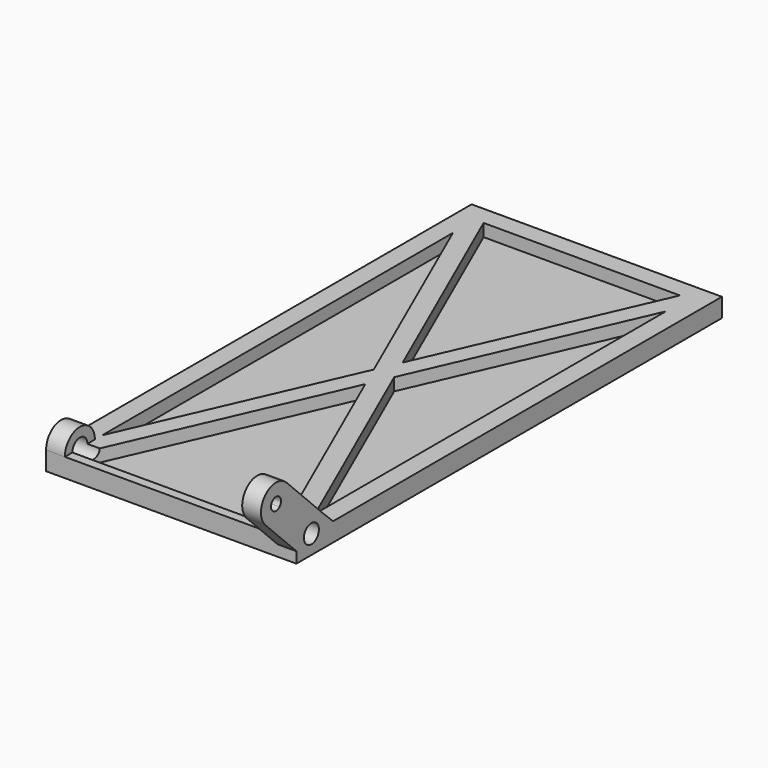
from build123d import *

# Parameters (mm, degrees)
F0_W      = 40
F0_H      = 85
F1_DEPTH  = 1
F2_W      = 3
F2_H      = 3
F3_DEPTH  = 2
F5_DEPTH  = 3
F7_DEPTH  = 3
F9_R      = 1.5
F10_DEPTH = 45


with BuildPart() as f1:
    # F0 (on Top) → F1 (new body)
    with BuildSketch(Plane.XY):
        Rectangle(F0_W, F0_H)
    extrude(amount=F1_DEPTH)

    # F2 (on face) → F3 (join)
    with BuildSketch(Plane.XY.offset(1)):
        Polygon((-17, -42.5), (17, -42.5), (15.6843836329, -39.5), (-15.6843836329, -39.5), align=None)
        Polygon((-17, -39.5), (-17, -42.5), (-15.6843836329, -39.5), align=None)
        with Locations((-18.5, -41)):
            Rectangle(F2_W, F2_H)
        Polygon((15.6843836329, -39.5), (17, -42.5), (17, -39.5), align=None)
        with Locations((18.5, -41)):
            Rectangle(F2_W, F2_H)
        Polygon((17, -35.0301999523), (17, -39.5), (20, -39.5), (20, 39.5), (17, 39.5), (17, 35.0301999523), align=None)
        Polygon((15.6843836329, -39.5), (17, -39.5), (17, -35.0301999523), (1.6378985336, 0), (0, -3.7349000238), align=None)
        Polygon((-15.6843836329, -39.5), (0, -3.7349000238), (-1.6378985336, 0), (-17, -35.0301999523), (-17, -39.5), align=None)
        Polygon((-20, -39.5), (-17, -39.5), (-17, -35.0301999523), (-17, 35.0301999523), (-17, 39.5), (-20, 39.5), align=None)
        Polygon((-1.6378985336, 0), (0, -3.7349000238), (1.6378985336, 0), (0, 3.7349000238), align=None)
        Polygon((-17, 35.0301999523), (-1.6378985336, 0), (0, 3.7349000238), (-15.6843836329, 39.5), (-17, 39.5), align=None)
        Polygon((1.6378985336, 0), (17, 35.0301999523), (17, 39.5), (15.6843836329, 39.5), (0, 3.7349000238), align=None)
        with Locations((-18.5, 41)):
            Rectangle(F2_W, F2_H)
        Polygon((-17, 39.5), (-15.6843836329, 39.5), (-17, 42.5), align=None)
        Polygon((15.6843836329, 39.5), (17, 42.5), (-17, 42.5), (-15.6843836329, 39.5), align=None)
        Polygon((15.6843836329, 39.5), (17, 39.5), (17, 42.5), align=None)
        with Locations((18.5, 41)):
            Rectangle(F2_W, F2_H)
    extrude(amount=F3_DEPTH)

    # F4 (on face) → F5 (join)
    with BuildSketch(Plane.YZ.offset(20)):
        with BuildLine():
            ThreePointArc((-42.5, 3), (-42.2716385975, 4.1480502971), (-41.6213203436, 5.1213203436))
            Line((-41.6213203436, 5.1213203436), (-44.4490675498, 7.9490675498))
            ThreePointArc((-44.4490675498, 7.9490675498), (-46.5442111918, 7.0702264387), (-48.6547486938, 7.9114279791))
            Line((-48.6547486938, 7.9114279791), (-42.5, 1.7572743533))
            Line((-42.5, 1.7572743533), (-42.5, 3))
        make_face()
        with BuildLine():
            Line((-39.5, 3), (-36.5, 3))
            ThreePointArc((-36.5, 3), (-36.7387500509, 4.1728165749), (-37.4169991456, 5.1589598052))
            ThreePointArc((-37.4169991456, 5.1589598052), (-39.5268566208, 5.9998797846), (-41.6213203436, 5.1213203436))
            Line((-41.6213203436, 5.1213203436), (-39.5, 3))
        make_face()
        with BuildLine():
            Line((-42.5, 3), (-39.5, 3))
            Line((-39.5, 3), (-41.6213203436, 5.1213203436))
            ThreePointArc((-41.6213203436, 5.1213203436), (-42.2716385975, 4.1480502971), (-42.5, 3))
        make_face()
        with BuildLine():
            ThreePointArc((-37.4169991456, 5.1589598052), (-36.7387500509, 4.1728165749), (-36.5, 3))
            Line((-36.5, 3), (-35.1793104616, 3))
            Line((-35.1793104616, 3), (-37.4169991456, 5.1589598052))
        make_face()
        with BuildLine():
            ThreePointArc((-41.6213203436, 5.1213203436), (-39.5268566208, 5.9998797846), (-37.4169991456, 5.1589598052))
            Line((-37.4169991456, 5.1589598052), (-44.3843033436, 12.1262640032))
            ThreePointArc((-44.3843033436, 12.1262640032), (-43.7810708304, 11.1763673496), (-43.5701062619, 10.0710678119))
            ThreePointArc((-43.5701062619, 10.0710678119), (-43.798540858, 8.9226495455), (-44.4490675498, 7.9490675498))
            Line((-44.4490675498, 7.9490675498), (-41.6213203436, 5.1213203436))
        make_face()
        with BuildLine():
            ThreePointArc((-43.5701062619, 10.0710678119), (-43.7810708304, 11.1763673496), (-44.3843033436, 12.1262640032))
            Line((-44.3843033436, 12.1262640032), (-44.4121080066, 12.1540686663))
            Line((-44.4121080066, 12.1540686663), (-45.8270022514, 10.7391744215))
            ThreePointArc((-45.8270022514, 10.7391744215), (-45.6372408578, 10.4287928736), (-45.5710678119, 10.0710678119))
            ThreePointArc((-45.5710678119, 10.0710678119), (-45.6471882794, 9.6883843795), (-45.8639610307, 9.3639610307))
            Line((-45.8639610307, 9.3639610307), (-44.4490675498, 7.9490675498))
            ThreePointArc((-44.4490675498, 7.9490675498), (-43.798540858, 8.9226495455), (-43.5701062619, 10.0710678119))
        make_face()
        with BuildLine():
            ThreePointArc((-48.6547486938, 7.9114279791), (-46.5442111918, 7.0702264387), (-44.4490675498, 7.9490675498))
            Line((-44.4490675498, 7.9490675498), (-45.8639610307, 9.3639610307))
            ThreePointArc((-45.8639610307, 9.3639610307), (-46.5442025706, 9.0714287476), (-47.2391744215, 9.3270022514))
            Line((-47.2391744215, 9.3270022514), (-48.6547486938, 7.9114279791))
        make_face()
        with BuildLine():
            Line((-44.4121080066, 12.1540686663), (-44.3843033436, 12.1262640032))
            ThreePointArc((-44.3843033436, 12.1262640032), (-48.6791160167, 12.2069289943), (-48.6547486938, 7.9114279791))
            Line((-48.6547486938, 7.9114279791), (-47.2391744215, 9.3270022514))
            ThreePointArc((-47.2391744215, 9.3270022514), (-47.2781745931, 10.7781745931), (-45.8270022514, 10.7391744215))
            Line((-45.8270022514, 10.7391744215), (-44.4121080066, 12.1540686663))
        make_face()
    extrude(amount=-F5_DEPTH)

    # F6 (on face) → F7 (join)
    with BuildSketch(Plane(origin=(-20, 0, 0), x_dir=(0, -1, 0), z_dir=(-1, 0, 0))):
        with BuildLine():
            Line((36.5, 3), (42.5, 3))
            ThreePointArc((42.5, 3), (39.5, 6), (36.5, 3))
        make_face()
        with BuildLine():
            ThreePointArc((39.5000000598, 0), (41.6213203647, 0.8786796776), (42.5, 3))
            Line((42.5, 3), (36.5, 3))
            ThreePointArc((36.5, 3), (37.3786796776, 0.8786796353), (39.5000000598, 0))
        make_face()
    extrude(amount=-F7_DEPTH)

    # F8: union 

    # F9 (on face) → F10 (cut)
    with BuildSketch(Plane(origin=(-20, 0, 0), x_dir=(0, -1, 0), z_dir=(-1, 0, 0))):
        with Locations((39.5, 3)):
            Circle(F9_R)
    extrude(amount=-F10_DEPTH, mode=Mode.SUBTRACT)


solid = f1.part
